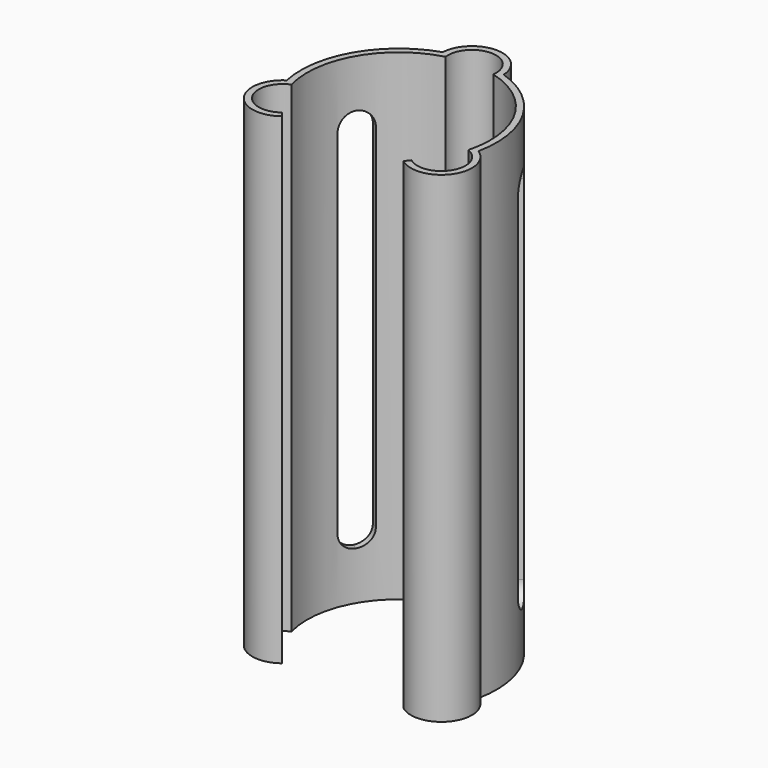
from build123d import *

# Parameters (mm, degrees)
F1_DEPTH = 150
F4_DEPTH = 14.6
F7_DEPTH = 25


with BuildPart() as f1:
    # F0 (on Top) → F1 (new body)
    with BuildSketch(Plane.XY):
        with BuildLine():
            ThreePointArc((-20.1233408974, -5.9455809682), (-31.1901518255, -3.7500670345), (-27.5583376919, 6.9319043027))
            ThreePointArc((-27.5583376919, 6.9319043027), (-24.6952207253, 28.5156271448), (-7.4348638898, 41.787198732))
            ThreePointArc((-7.4348638898, 41.787198732), (0, 50.2735044354), (7.4348638898, 41.787198732))
            ThreePointArc((7.4348638898, 41.787198732), (24.6952207253, 28.5156271448), (27.5583376919, 6.9319043027))
            ThreePointArc((27.5583376919, 6.9319043027), (31.1901518255, -3.7500670345), (20.1233408974, -5.9455809682))
            Line((20.1233408974, -5.9455809682), (18.9042318034, -7.5310692264))
            ThreePointArc((18.9042318034, -7.5310692264), (32.4530777326, -5.4829034184), (29.8611497399, 7.9725088187))
            ThreePointArc((29.8611497399, 7.9725088187), (26.4272766932, 29.5156182068), (9.4874750724, 43.2611690236))
            ThreePointArc((9.4874750724, 43.2611690236), (0, 52.2735044354), (-9.4874750724, 43.2611690236))
            ThreePointArc((-9.4874750724, 43.2611690236), (-26.4272766932, 29.5156182068), (-29.8611497399, 7.9725088187))
            ThreePointArc((-29.8611497399, 7.9725088187), (-32.4530777326, -5.4829034184), (-18.9042318034, -7.5310692264))
            Line((-18.9042318034, -7.5310692264), (-20.1233408974, -5.9455809682))
        make_face()
    extrude(amount=F1_DEPTH)

    # F3 (on 3pt) → F4 (cut)
    with BuildSketch(Plane(origin=(25.8481727674, 14.9232716588, 0), x_dir=(0.499995531, -0.8660279839, 0), z_dir=(-0.8660279839, -0.499995531, 0))):
        with BuildLine():
            Line((-7.3478311295, 20), (-7.3478311295, 130))
            ThreePointArc((-7.3478311295, 130), (-8.8122972235, 133.5355339059), (-12.3478311295, 135))
            ThreePointArc((-12.3478311295, 135), (-15.8833650354, 133.5355339059), (-17.3478311295, 130))
            Line((-17.3478311295, 130), (-17.3478311295, 20))
            ThreePointArc((-17.3478311295, 20), (-15.8833650354, 16.4644660941), (-12.3478311295, 15))
            ThreePointArc((-12.3478311295, 15), (-8.8122972235, 16.4644660941), (-7.3478311295, 20))
        make_face()
    extrude(amount=-F4_DEPTH, mode=Mode.SUBTRACT)

    # F6 (on 3pt) → F7 (cut)
    with BuildSketch(Plane(origin=(-25.8481727674, 14.9232716588, 0), x_dir=(-0.499995531, -0.8660279839, 0), z_dir=(-0.8660279839, 0.499995531, 0))):
        with BuildLine():
            ThreePointArc((-12.3478310445, 135), (-15.8833649505, 133.5355339059), (-17.3478310445, 130))
            Line((-17.3478310445, 130), (-17.3478310445, 20))
            ThreePointArc((-17.3478310445, 20), (-15.8833649505, 16.4644660941), (-12.3478310445, 15))
            ThreePointArc((-12.3478310445, 15), (-8.8122971386, 16.4644660941), (-7.3478310445, 20))
            Line((-7.3478310445, 20), (-7.3478310445, 130))
            ThreePointArc((-7.3478310445, 130), (-8.8122971386, 133.5355339059), (-12.3478310445, 135))
        make_face()
    extrude(amount=F7_DEPTH, mode=Mode.SUBTRACT)


solid = f1.part
